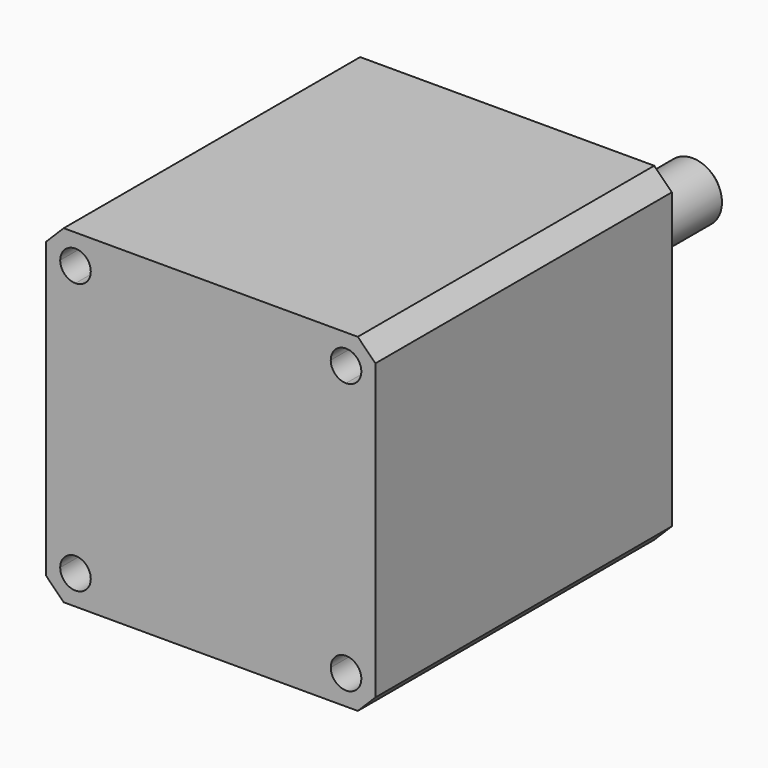
from build123d import *

# Parameters (mm, degrees)
F0_W      = 28
F0_H      = 28
F1_DEPTH  = 31.5
F2_R      = 11
F3_DEPTH  = 1.5
F4_R      = 2.5
F5_DEPTH  = 18.5
F6_SIZE   = 1.5
F7_SIZE   = 0.3
F8_R      = 1.49999
F10_DEPTH = 31.5


# Not quite as in the source:
# - a fillet or chamfer is up to 0.001 mm smaller than in the source, because OpenCascade refuses the exact size


with BuildPart() as f1:
    # F0 (on Front) → F1 (new body)
    with BuildSketch(Plane.XZ):
        Rectangle(F0_W, F0_H)
    extrude(amount=-F1_DEPTH)

    # F2 (on face) → F3 (join)
    with BuildSketch(Plane(origin=(0, 31.5, 0), x_dir=(-1, 0, 0), z_dir=(0, 1, 0))):
        Circle(F2_R)
    extrude(amount=F3_DEPTH)

    # F4 (on face) → F5 (join)
    with BuildSketch(Plane(origin=(0, 33, 0), x_dir=(-1, 0, 0), z_dir=(0, 1, 0))):
        Circle(F4_R)
    extrude(amount=F5_DEPTH)

    # F6
    f6_edges = [f1.edges().sort_by_distance(p)[0] for p in [
        (14, 15.75, 14),
        (14, 15.75, -14),
        (-14, 15.75, -14),
        (-14, 15.75, 14),
    ]]
    chamfer(f6_edges, length=F6_SIZE)

    # F7
    f7_edges = [f1.edges().sort_by_distance(p)[0] for p in [
        (2.5, 51.5, 0),
    ]]
    chamfer(f7_edges, length=F7_SIZE)

    # F8 (radius 1.5 in the source; OpenCascade refuses exactly that, so slightly less here)
    f8_edges = [f1.edges().sort_by_distance(p)[0] for p in [
        (11, 33, 0),
    ]]
    fillet(f8_edges, radius=F8_R)

    # F9 (on face) → F10 (cut)
    with BuildSketch(Plane(origin=(0, 31.5, 0), x_dir=(-1, 0, 0), z_dir=(0, 1, 0))):
        with BuildLine():
            Line((-11.5, -11.5), (-11.5, -10.2))
            ThreePointArc((-11.5, -10.2), (-12.4192388155, -12.4192388155), (-10.2, -11.5))
            Line((-10.2, -11.5), (-11.5, -11.5))
        make_face()
        with BuildLine():
            ThreePointArc((-10.2, -11.5), (-10.5807611845, -10.5807611845), (-11.5, -10.2))
            Line((-11.5, -10.2), (-11.5, -11.5))
            Line((-11.5, -11.5), (-10.2, -11.5))
        make_face()
        with BuildLine():
            ThreePointArc((12.8, -11.5), (12.4192388155, -10.5807611845), (11.5, -10.2))
            Line((11.5, -10.2), (11.5, -11.5))
            Line((11.5, -11.5), (10.2, -11.5))
            ThreePointArc((10.2, -11.5), (11.5, -12.8), (12.8, -11.5))
        make_face()
        with BuildLine():
            Line((11.5, -11.5), (11.5, -10.2))
            ThreePointArc((11.5, -10.2), (10.5807611845, -10.5807611845), (10.2, -11.5))
            Line((10.2, -11.5), (11.5, -11.5))
        make_face()
        with BuildLine():
            Line((11.5, 11.5), (10.2, 11.5))
            ThreePointArc((10.2, 11.5), (10.5807611845, 10.5807611845), (11.5, 10.2))
            Line((11.5, 10.2), (11.5, 11.5))
        make_face()
        with BuildLine():
            ThreePointArc((12.8, 11.5), (11.5, 12.8), (10.2, 11.5))
            Line((10.2, 11.5), (11.5, 11.5))
            Line((11.5, 11.5), (11.5, 10.2))
            ThreePointArc((11.5, 10.2), (12.4192388155, 10.5807611845), (12.8, 11.5))
        make_face()
        with BuildLine():
            ThreePointArc((-11.5, 10.2), (-10.5807611845, 10.5807611845), (-10.2, 11.5))
            Line((-10.2, 11.5), (-11.5, 11.5))
            Line((-11.5, 11.5), (-11.5, 10.2))
        make_face()
        with BuildLine():
            Line((-11.5, 11.5), (-10.2, 11.5))
            ThreePointArc((-10.2, 11.5), (-12.4192388155, 12.4192388155), (-11.5, 10.2))
            Line((-11.5, 10.2), (-11.5, 11.5))
        make_face()
    extrude(amount=-F10_DEPTH, mode=Mode.SUBTRACT)


solid = f1.part
